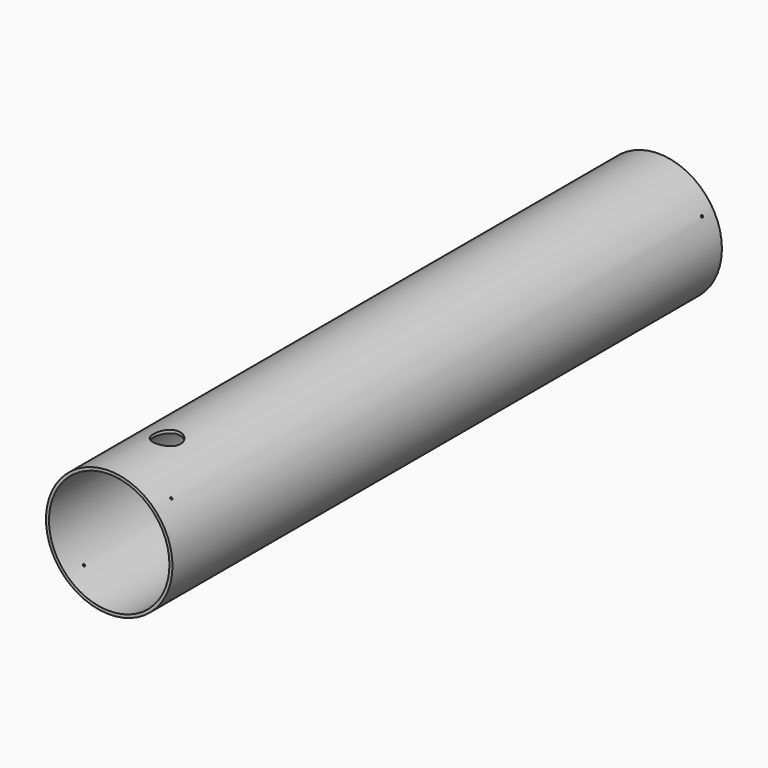
from build123d import *

# Parameters (mm, degrees)
F0_R             = 133.35
F0_R_2           = 127
F2_DEPTH         = 1447.8
F5_D             = 57.15
F5_DEPTH         = 12.7
F5_START         = 3.0975841
F5_TIP           = 17.1695921887
F7_R             = 2.38125
F8_DEPTH         = 25.4
F8_COPIES_COUNT  = 4
F10_R            = 2.38125
F11_DEPTH        = 25.4
F11_COPIES_COUNT = 3


# Not quite as in the source:
# - a pattern or mirror of a feature is missing from the dataset's text; its kind, count and spacing are read off the source's solid


with BuildPart() as f2:
    # F0 (on Front) → F2 (new body)
    with BuildSketch(Plane.XZ):
        Circle(F0_R)
        Circle(F0_R_2, mode=Mode.SUBTRACT)
    extrude(amount=-F2_DEPTH)

    # F5
    # its depths count from where the whole tool has entered the part; down to there all is cleared
    with Locations(Plane.XY.offset(133.35).offset(-F5_START)):
        with Locations((0, 152.4)):
            Hole(F5_D / 2, depth=F5_DEPTH)
            with Locations((0, 0, -(F5_DEPTH + F5_TIP / 2))):  # 118° drill point
                Cone(0, F5_D / 2, F5_TIP, mode=Mode.SUBTRACT)

    # F7 (on line) → F8 (cut)
    with BuildSketch(Plane(origin=(-94.2926892712, 0, 94.2926892712), x_dir=(0, -1, 0), z_dir=(-0.7071067812, 0, 0.7071067812))):
        with Locations((-45.72, 0)):
            Circle(F7_R)
    f8 = extrude(amount=-F8_DEPTH, mode=Mode.SUBTRACT)

    # F8_copies: F8 ×4 about axis
    f8_copies_axis = Axis((0, 0, 0), (0, 1, 0))
    for i in range(1, F8_COPIES_COUNT):
        add(f8.rotate(f8_copies_axis, i * 360 / F8_COPIES_COUNT), mode=Mode.SUBTRACT)

    # F10 (on line) → F11 (cut)
    with BuildSketch(Plane(origin=(-115.4844875947, 0, 66.675), x_dir=(0, -1, 0), z_dir=(-0.8660254038, 0, 0.5))):
        with Locations((-1417.447, 0)):
            Circle(F10_R)
    f11 = extrude(amount=-F11_DEPTH, mode=Mode.SUBTRACT)

    # F11_copies: F11 ×3 about axis
    f11_copies_axis = Axis((0, 0, 0), (0, 1, 0))
    for i in range(1, F11_COPIES_COUNT):
        add(f11.rotate(f11_copies_axis, i * 360 / F11_COPIES_COUNT), mode=Mode.SUBTRACT)


solid = f2.part
